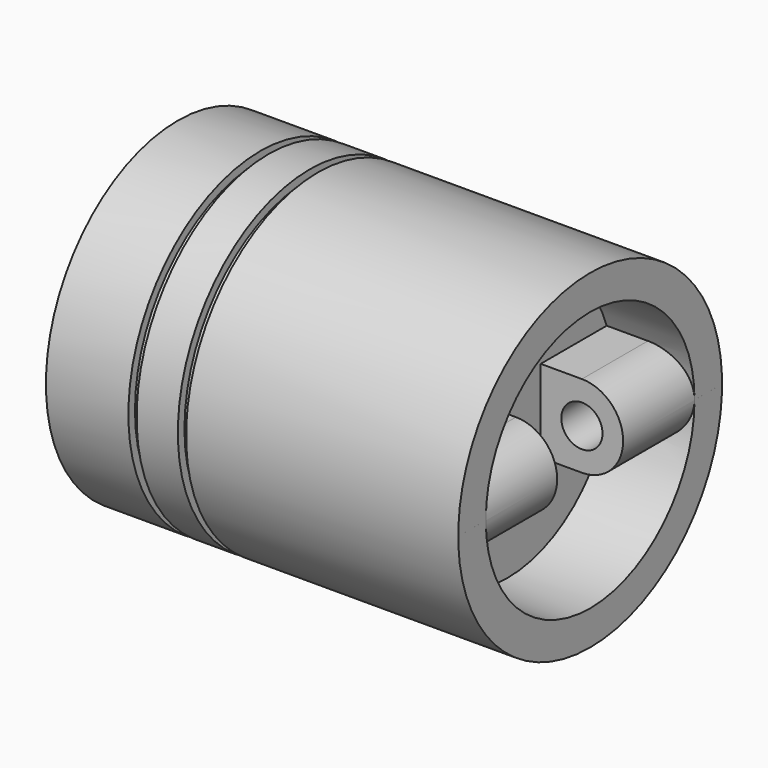
from build123d import *

# Parameters (mm, degrees)
F2_R          = 40.1855244707
F3_DEPTH      = 25.4
F4_R          = 6.35
F5_DEPTH      = 48.26
F5_DEPTH_BACK = 48.26
F6_DEPTH      = 12.7
F6_DEPTH_BACK = 12.7


# Not quite as in the source:
# - ends of sketch curves that miss each other by under 0.0002 mm in the source are joined


with BuildPart() as f1:
    # F0 (on Front) → F1 (revolve)
    with BuildSketch(Plane.XZ):
        Polygon((0, 50.8), (0, 0), (127, 0), (127, 50.8), (43.18, 50.8), (43.18, 48.26), (40.64, 48.26), (40.64, 50.8), (27.94, 50.8), (27.94, 48.26), (25.4, 48.26), (25.4, 50.8), align=None)
    revolve(axis=Axis((-13.3472196758, 0, 0), (1, 0, 0)))

    # F2 (on face) → F3 (cut)
    with BuildSketch(Plane.YZ.offset(127)):
        Circle(F2_R)
    extrude(amount=-F3_DEPTH, mode=Mode.SUBTRACT)

    # F4 (on Front) → F5 (join, two sides)
    with BuildSketch(Plane.XZ) as f5_sk:
        with BuildLine():
            Line((101.6, -12.7), (114.3, -12.7))
            ThreePointArc((114.3, -12.7), (127.0000011214, 0), (114.3, 12.7000011214))
            Line((114.3, 12.7000011214), (101.6, 12.7))
            Line((101.6, 12.7), (101.6, -12.7))
        make_face()
        with Locations((114.3, 0)):
            Circle(F4_R, mode=Mode.SUBTRACT)
    extrude(amount=F5_DEPTH)
    extrude(f5_sk.sketch, amount=-F5_DEPTH_BACK)

    # F4 (on Front) → F6 (cut, two sides)
    with BuildSketch(Plane.XZ) as f6_sk:
        with BuildLine():
            Line((101.6, -12.7), (114.3, -12.7))
            ThreePointArc((114.3, -12.7), (127.0000011214, 0), (114.3, 12.7000011214))
            Line((114.3, 12.7000011214), (101.6, 12.7))
            Line((101.6, 12.7), (101.6, -12.7))
        make_face()
        with Locations((114.3, 0)):
            Circle(F4_R, mode=Mode.SUBTRACT)
    extrude(amount=-F6_DEPTH, mode=Mode.SUBTRACT)
    extrude(f6_sk.sketch, amount=F6_DEPTH_BACK, mode=Mode.SUBTRACT)

    # F7 (on Front) → F8 (revolve, cut)
    with BuildSketch(Plane.XZ):
        Polygon((0, 50.5328811705), (0, 0), (9.8897889256, 0), align=None)
    revolve(axis=Axis((4.9448944628, 0, 0), (-1, 0, 0)), mode=Mode.SUBTRACT)


solid = f1.part
